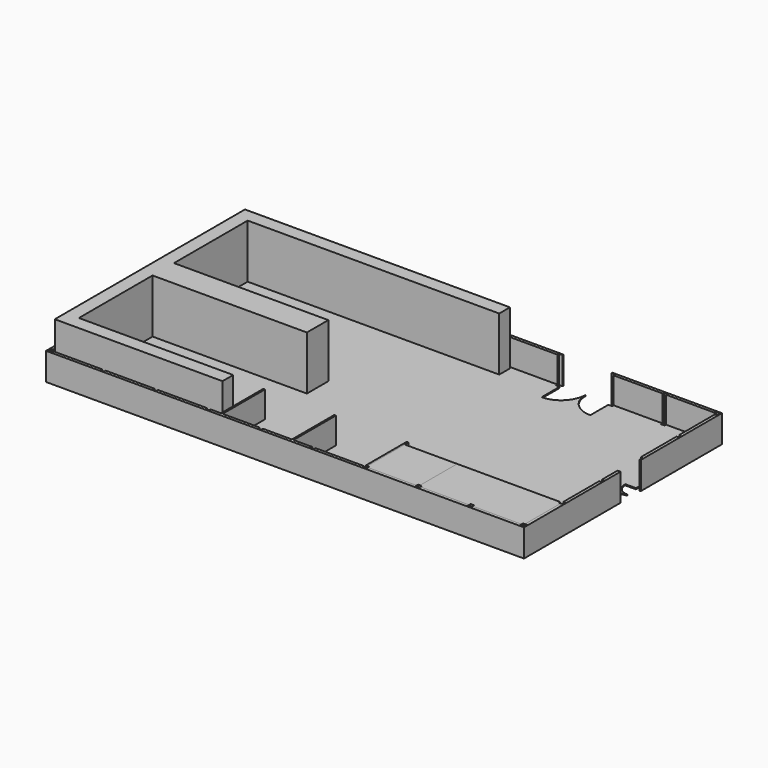
from build123d import *

# Parameters (mm, degrees)
F0_W     = 4500
F0_H     = 1300
F0_W_2   = 6308.3334
F0_H_2   = 4815
F0_H_3   = 150
F0_W_3   = 150
F0_W_4   = 6458.3334
F1_DEPTH = 100
F0_W_5   = 1220
F0_H_4   = 2440
F0_H_5   = 510
F0_H_6   = 1220
F0_W_6   = 14060
F2_DEPTH = 5000
F3_DEPTH = 2500
F4_DEPTH = 2500
F5_DEPTH = 2500
F6_DEPTH = 2500


with BuildPart() as f1:
    # F0 (on Top) → F1 (new body)
    with BuildSketch(Plane.XY):
        with BuildLine():
            ThreePointArc((33274.4446, 19781.1111), (31705.4532121104, 20431.0086121104), (31055.5557, 22000))
            ThreePointArc((31055.5557, 22000), (30405.6581878896, 20431.0086121104), (28836.6668, 19781.1111))
            Line((28836.6668, 19781.1111), (28836.6668, 21830))
            Line((28836.6668, 21830), (28496.6668, 21830))
            Line((28496.6668, 21830), (28496.6668, 22000))
            Line((28496.6668, 22000), (24058.889, 22000))
            Line((24058.889, 22000), (24058.889, 21830))
            Line((24058.889, 21830), (24310, 21830))
            Line((24310, 21830), (24310, 20610))
            Line((24310, 20610), (23090, 20610))
            Line((23090, 20610), (21870, 20610))
            Line((21870, 20610), (16670, 20610))
            Line((16670, 20610), (15450, 20610))
            Line((15450, 20610), (14230, 20610))
            Line((14230, 20610), (9030, 20610))
            Line((9030, 20610), (7810, 20610))
            Line((7810, 20610), (6590, 20610))
            Line((6590, 20610), (1390, 20610))
            Line((1390, 20610), (1390, 12730))
            Line((1390, 12730), (1390, 12220))
            Line((1390, 12220), (15450, 12220))
            Line((15450, 12220), (15450, 9780))
            Line((15450, 9780), (15600, 9780))
            Line((15600, 9780), (21908.3334, 9780))
            Line((21908.3334, 9780), (22058.3334, 9780))
            Line((22058.3334, 9780), (28516.6668, 9780))
            Line((28516.6668, 9780), (28666.6668, 9780))
            Line((28666.6668, 9780), (28666.6668, 4815))
            Line((28666.6668, 4815), (28666.6668, 4400))
            Line((28666.6668, 4400), (33444.4446, 4400))
            Line((33444.4446, 4400), (42830, 4400))
            Line((42830, 4400), (42830, 4570))
            Line((42830, 4570), (43000, 4570))
            Line((43000, 4570), (43000, 8630))
            Line((43000, 8630), (42830, 8630))
            Line((42830, 8630), (42830, 8970))
            Line((42830, 8970), (43000, 8970))
            Line((43000, 8970), (43000, 10730))
            Line((43000, 10730), (41850, 10730))
            ThreePointArc((41850, 10730), (42186.8272016355, 11543.1727983645), (43000, 11880))
            ThreePointArc((43000, 11880), (42186.8272016355, 12216.8272016355), (41850, 13030))
            Line((41850, 13030), (42830, 13030))
            Line((42830, 13030), (42830, 13370))
            Line((42830, 13370), (43000, 13370))
            Line((43000, 13370), (43000, 17430))
            Line((43000, 17430), (42830, 17430))
            Line((42830, 17430), (42830, 17770))
            Line((42830, 17770), (43000, 17770))
            Line((43000, 17770), (43000, 21830))
            Line((43000, 21830), (42830.0002, 21830))
            Line((42830.0002, 21830), (42830.0002, 22000))
            Line((42830.0002, 22000), (38392.2224, 22000))
            Line((38392.2224, 22000), (38392.2224, 21830))
            Line((38392.2224, 21830), (38052.2224, 21830))
            Line((38052.2224, 21830), (38052.2224, 22000))
            Line((38052.2224, 22000), (33614.4446, 22000))
            Line((33614.4446, 22000), (33614.4446, 21830))
            Line((33614.4446, 21830), (33274.4446, 21830))
            Line((33274.4446, 21830), (33274.4446, 19781.1111))
        make_face()
        with Locations((3865.0875091553, 17252.7908325195)):
            Rectangle(F0_W, F0_H, mode=Mode.SUBTRACT)
        with Locations((3865.0875091553, 17252.7908325195)):
            Rectangle(F0_W, F0_H)
        Polygon((33444.4446, 170), (33444.4446, 4400), (28666.6668, 4400), (28666.6668, 170), (28836.6668, 170), (28836.6668, 0), (33274.4446, 0), (33274.4446, 170), align=None)
        Polygon((43000.0001922727, 170), (43000.0000077273, 4230), (42830, 4230), (42830, 4400), (33444.4446, 4400), (33444.4446, 170), (33614.4446, 170), (33614.4446, 0), (38052.2224, 0), (38052.2224, 170), (38392.2224, 170), (38392.2224, 0), (42830.0002, 0), (42830.0002, 170), align=None)
        Polygon((28496.6668, 170), (28516.6668, 170), (28516.6668, 4400), (28516.6668, 4815), (22058.3334, 4815), (22058.3334, 0), (23718.889, 0), (23718.889, 170), (24058.889, 170), (24058.889, 0), (28496.6668, 0), align=None)
        Polygon((21908.3334, 0), (21908.3334, 4815), (15600, 4815), (15600, 0), (18941.1112, 0), (18941.1112, 170), (19281.1112, 170), (19281.1112, 0), align=None)
        Polygon((15450, 9780), (1390, 9780), (1390, 9270), (1390, 1390), (6590, 1390), (7810, 1390), (9030, 1390), (14230, 1390), (15450, 1390), (15450, 4815), (15450, 9270), align=None)
        with Locations((18754.1667, 7222.5)):
            Rectangle(F0_W_2, F0_H_2)
        Polygon((15600, 9780), (15450, 9780), (15450, 9270), (15450, 4815), (15600, 4815), (15600, 9630), align=None)
        with Locations((18754.1667, 9705)):
            Rectangle(F0_W_2, F0_H_3)
        with Locations((21983.3334, 9705)):
            Rectangle(F0_W_3, F0_H_3)
        with Locations((21983.3334, 7222.5)):
            Rectangle(F0_W_3, F0_H_2)
        with Locations((25287.5001, 9705)):
            Rectangle(F0_W_4, F0_H_3)
        with Locations((25287.5001, 7222.5)):
            Rectangle(F0_W_4, F0_H_2)
        Polygon((28516.6668, 4815), (28666.6668, 4815), (28666.6668, 9780), (28516.6668, 9780), (28516.6668, 9630), align=None)
    extrude(amount=F1_DEPTH)

    # F0 (on Top) → F3 (join)
    with BuildSketch(Plane.XY):
        with Locations((21983.3334, 2407.5)):
            Rectangle(F0_W_3, F0_H_2)
        Polygon((15600, 4815), (15450, 4815), (15450, 1390), (15450, 170), (15450, 0), (15600, 0), align=None)
        Polygon((28666.6668, 170), (28666.6668, 4400), (28666.6668, 4815), (28516.6668, 4815), (28516.6668, 4400), (28516.6668, 170), align=None)
    extrude(amount=F3_DEPTH)

    # F0 (on Top) → F4 (join)
    with BuildSketch(Plane.XY):
        Polygon((24058.889, 22000), (28496.6668, 22000), (28496.6668, 22170), (28836.6668, 22170), (28836.6668, 22270), (-270, 22270), (-270, -270), (43270.0002, -270), (43270.0002, 10730), (43000, 10730), (43000, 8970), (43170, 8970), (43170, 8630), (43000, 8630), (43000, 4570), (43170, 4570), (43170, 4230), (43000.0000077273, 4230), (43000.0001922727, 170), (43170.0002, 170), (43170.0002, -170), (42830.0002, -170), (42830.0002, 0), (38392.2224, 0), (38392.2224, -170), (38052.2224, -170), (38052.2224, 0), (33614.4446, 0), (33614.4446, -170), (33274.4446, -170), (33274.4446, 0), (28836.6668, 0), (28836.6668, -170), (28496.6668, -170), (28496.6668, 0), (24058.889, 0), (24058.889, -170), (23718.889, -170), (23718.889, 0), (22058.3334, 0), (21908.3334, 0), (19281.1112, 0), (19281.1112, -170), (18941.1112, -170), (18941.1112, 0), (15600, 0), (15450, 0), (14503.3334, 0), (14503.3334, -170), (14163.3334, -170), (14163.3334, 0), (9725.5556, 0), (9725.5556, -170), (9385.5556, -170), (9385.5556, 0), (4947.7778, 0), (4947.7778, -170), (4607.7778, -170), (4607.7778, 0), (170, 0), (170, -170), (-170, -170), (-170, 170), (0, 170), (0, 4230), (-170, 4230), (-170, 4570), (0, 4570), (0, 8630), (-170, 8630), (-170, 8970), (0, 8970), (0, 9780), (0, 12220), (0, 13030), (-170, 13030), (-170, 13370), (0, 13370), (0, 17430), (-170, 17430), (-170, 17770), (0, 17770), (0, 21830), (-170, 21830), (-170, 22170), (170, 22170), (170, 22000), (4607.7778, 22000), (4607.7778, 22170), (4947.7778, 22170), (4947.7778, 22000), (9385.5556, 22000), (9385.5556, 22170), (9725.5556, 22170), (9725.5556, 22000), (14163.3334, 22000), (14163.3334, 22170), (14503.3334, 22170), (14503.3334, 22000), (18941.1112, 22000), (18941.1112, 22170), (19281.1112, 22170), (19281.1112, 22000), (23718.889, 22000), (23718.889, 22170), (24058.889, 22170), align=None)
        Polygon((33614.4446, 22170), (33614.4446, 22000), (38052.2224, 22000), (38052.2224, 22170), (38392.2224, 22170), (38392.2224, 22000), (42830.0002, 22000), (42830.0002, 22170), (43170.0002, 22170), (43170.0002, 21830), (43000, 21830), (43000, 17770), (43170, 17770), (43170, 17430), (43000, 17430), (43000, 13370), (43170, 13370), (43170, 13030), (43270.0002, 13030), (43270.0002, 22270), (33274.4446, 22270), (33274.4446, 22170), align=None)
    extrude(amount=F4_DEPTH)


with BuildPart() as f2:
    # F0 (on Top) → F2 (new body)
    with BuildSketch(Plane.XY):
        Polygon((1390, 21830), (170, 21830), (170, 17770), (170, 17430), (170, 13370), (170, 13030), (170, 12730), (1390, 12730), (1390, 20610), align=None)
        Polygon((15450, 21830), (14503.3334, 21830), (14230, 21830), (14230, 20610), (15450, 20610), align=None)
        Polygon((15450, 170), (15450, 1390), (14230, 1390), (14230, 170), (14503.3334, 170), align=None)
        Polygon((1390, 1390), (1390, 9270), (170, 9270), (170, 8970), (170, 8630), (170, 4570), (170, 4230), (170, 170), (1390, 170), align=None)
        with Locations((780, 11000)):
            Rectangle(F0_W_5, F0_H_4)
        with Locations((780, 12475)):
            Rectangle(F0_W_5, F0_H_5)
        with Locations((780, 9525)):
            Rectangle(F0_W_5, F0_H_5)
        Polygon((6590, 21830), (4947.7778, 21830), (4607.7778, 21830), (1390, 21830), (1390, 20610), (6590, 20610), align=None)
        with Locations((7200, 21220)):
            Rectangle(F0_W_5, F0_H_6)
        with Locations((8420, 21220)):
            Rectangle(F0_W_5, F0_H_6)
        Polygon((14230, 21830), (14163.3334, 21830), (9725.5556, 21830), (9385.5556, 21830), (9030, 21830), (9030, 20610), (14230, 20610), align=None)
        with Locations((16060, 21220)):
            Rectangle(F0_W_5, F0_H_6)
        Polygon((21870, 21830), (19281.1112, 21830), (18941.1112, 21830), (16670, 21830), (16670, 20610), (21870, 20610), align=None)
        with Locations((22480, 21220)):
            Rectangle(F0_W_5, F0_H_6)
        Polygon((24310, 21830), (24058.889, 21830), (23718.889, 21830), (23090, 21830), (23090, 20610), (24310, 20610), align=None)
        Polygon((6590, 1390), (1390, 1390), (1390, 170), (4607.7778, 170), (4947.7778, 170), (6590, 170), align=None)
        with Locations((7200, 780)):
            Rectangle(F0_W_5, F0_H_6)
        with Locations((8420, 780)):
            Rectangle(F0_W_5, F0_H_6)
        Polygon((14230, 170), (14230, 1390), (9030, 1390), (9030, 170), (9385.5556, 170), (9725.5556, 170), (14163.3334, 170), align=None)
        with Locations((8420, 11000)):
            Rectangle(F0_W_6, F0_H_4)
    extrude(amount=F2_DEPTH)


with BuildPart() as f5:
    # F0 (on Top) → F5 (new body)
    with BuildSketch(Plane.XY):
        Polygon((33444.4446, 170), (33444.4446, 4400), (28666.6668, 4400), (28666.6668, 170), (28836.6668, 170), (28836.6668, 0), (33274.4446, 0), (33274.4446, 170), align=None)
    extrude(amount=F5_DEPTH)


with BuildPart() as f6:
    # F0 (on Top) → F6 (new body)
    with BuildSketch(Plane.XY):
        Polygon((43000.0001922727, 170), (43000.0000077273, 4230), (42830, 4230), (42830, 4400), (33444.4446, 4400), (33444.4446, 170), (33614.4446, 170), (33614.4446, 0), (38052.2224, 0), (38052.2224, 170), (38392.2224, 170), (38392.2224, 0), (42830.0002, 0), (42830.0002, 170), align=None)
    extrude(amount=F6_DEPTH)


solid = Compound([f1.part, f2.part, f5.part, f6.part])
